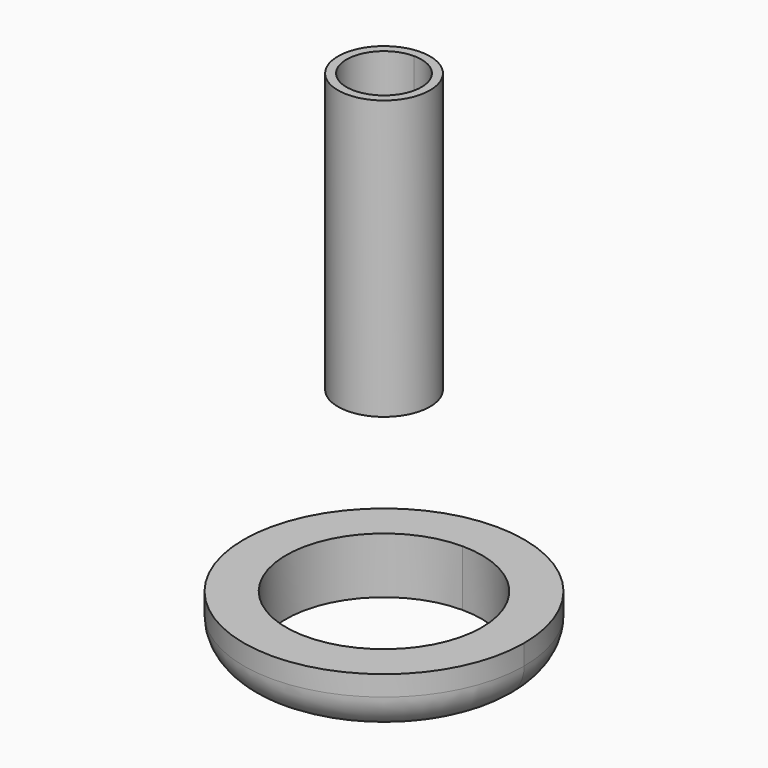
from build123d import *

# Parameters (mm, degrees)
F1_DEPTH = 7.9375
F3_R     = 6.5062989
F4_DEPTH = 39.37
F5_DEPTH = 25.4
F6_R     = 5.08


# Not quite as in the source:
# - the program builds the solid bodies; features that only make, move or delete a surface that nothing else refers to are left out


with BuildPart() as f1:
    # F0 (on Top) → F1 (new body)
    with BuildSketch(Plane.XY):
        with BuildLine():
            ThreePointArc((19.812, 0), (14.0091995489, 14.0091995489), (0, 19.812))
            ThreePointArc((0, 19.812), (-14.0091995489, -14.0091995489), (19.812, 0))
        make_face()
        with BuildLine():
            ThreePointArc((0, 13.8303), (9.7794989158, 9.7794989158), (13.8303, 0))
            ThreePointArc((13.8303, 0), (-9.7794989158, -9.7794989158), (0, 13.8303))
        make_face(mode=Mode.SUBTRACT)
    extrude(amount=F1_DEPTH)

    # F3 (on offset) → F5 (cut)
    with BuildSketch(Plane.XY.offset(33.02)):
        Circle(F3_R)
        with BuildLine():
            ThreePointArc((0, 5.294899345), (3.7440592325, 3.7440592325), (5.294899345, 0))
            ThreePointArc((5.294899345, 0), (-3.7440592325, -3.7440592325), (0, 5.294899345))
        make_face(mode=Mode.SUBTRACT)
    extrude(amount=-F5_DEPTH, mode=Mode.SUBTRACT)

    # F6
    f6_edges = [f1.edges().sort_by_distance(p)[0] for p in [
        (-19.812, 0, 0),
    ]]
    fillet(f6_edges, radius=F6_R)


with BuildPart() as f4:
    # F3 (on offset) → F4 (new body)
    with BuildSketch(Plane.XY.offset(33.02)):
        Circle(F3_R)
        with BuildLine():
            ThreePointArc((0, 5.294899345), (3.7440592325, 3.7440592325), (5.294899345, 0))
            ThreePointArc((5.294899345, 0), (-3.7440592325, -3.7440592325), (0, 5.294899345))
        make_face(mode=Mode.SUBTRACT)
    extrude(amount=F4_DEPTH)


solid = Compound([f1.part, f4.part])
